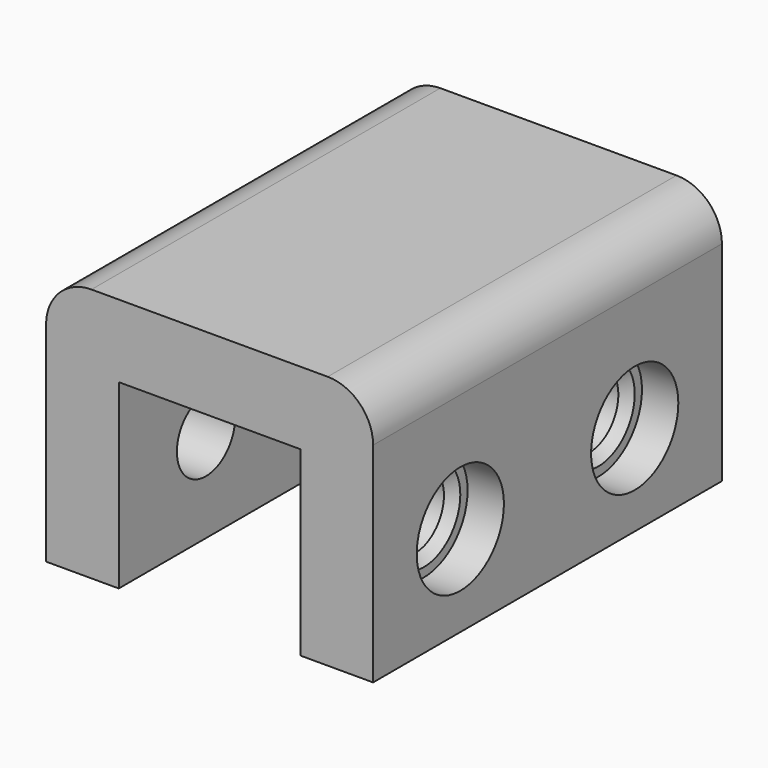
from build123d import *

# Parameters (mm, degrees)
F0_W     = 48
F0_H     = 28
F1_DEPTH = 36
F2_W     = 20
F2_H     = 48
F3_DEPTH = 20
F4_R     = 5
F5_R     = 4
F6_DEPTH = 36
F7_R     = 6
F8_DEPTH = 4
F9_SIZE  = 1


with BuildPart() as f1:
    # F0 (on Right) → F1 (new body)
    with BuildSketch(Plane.YZ):
        with Locations((-13.1489487588, -14)):
            Rectangle(F0_W, F0_H)
    extrude(amount=F1_DEPTH)

    # F2 (on face) → F3 (cut)
    with BuildSketch(Plane(origin=(0, 0, -28), x_dir=(1, 0, 0), z_dir=(0, 0, -1))):
        with Locations((18, 13.1489487588)):
            Rectangle(F2_W, F2_H)
    extrude(amount=-F3_DEPTH, mode=Mode.SUBTRACT)

    # F4
    f4_edges = [f1.edges().sort_by_distance(p)[0] for p in [
        (0, -13.148949, 0),
        (36, -13.148949, 0),
    ]]
    fillet(f4_edges, radius=F4_R)

    # F5 (on face) → F6 (cut)
    with BuildSketch(Plane.YZ.offset(36)):
        with Locations((46.8510512412, -18)):
            Circle(F5_R)
        with Locations((22.8510512412, -18)):
            Circle(F5_R)
        with Locations((-1.1489487588, -18)):
            Circle(F5_R)
        with Locations((-25.1489487588, -18)):
            Circle(F5_R)
    extrude(amount=-F6_DEPTH, mode=Mode.SUBTRACT)

    # F7 (on face) → F8 (cut)
    with BuildSketch(Plane.YZ.offset(36)):
        with Locations((-25.1489487588, -18)):
            Circle(F7_R)
        with Locations((-1.1489487588, -18)):
            Circle(F7_R)
        with Locations((22.8510512412, -18)):
            Circle(F7_R)
        with Locations((46.8510512412, -18)):
            Circle(F7_R)
    extrude(amount=-F8_DEPTH, mode=Mode.SUBTRACT)

    # F9
    f9_edges = [f1.edges().sort_by_distance(p)[0] for p in [
        (32, -29.148949, -18),
        (32, -5.148949, -18),
    ]]
    chamfer(f9_edges, length=F9_SIZE)


solid = f1.part
